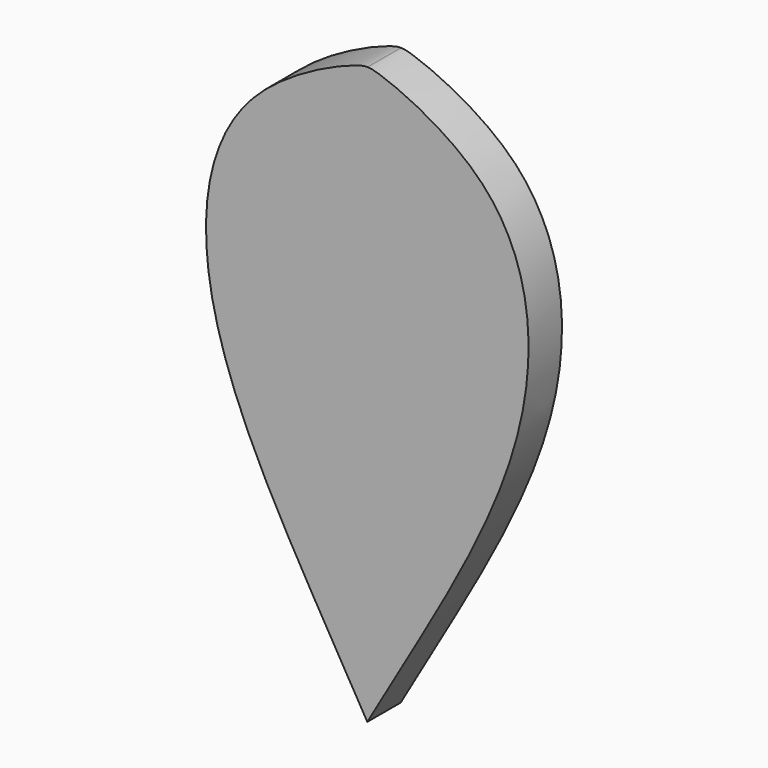
from build123d import *

# Parameters (mm, degrees)
F1_DEPTH = 5


with BuildPart() as f1:
    # F0 (on Front) → F1 (new body)
    with BuildSketch(Plane.XZ):
        with BuildLine():
            add(Edge.make_bspline(
                [(0, 0), (-7.8883632072, 13.8003130558), (-21.7462386942, 35.0909967896), (-18.519377881, 62.5951900227), (-0.8446341959, 69.1773688938), (-0.0343544445, 68.9731165883)],
                knots=[0, 0, 0, 0, 0.4098329947, 0.7231046582, 0.9651145636, 0.9651145636, 0.9651145636, 0.9651145636], degree=3))
            add(Edge.make_bspline(
                [(0, 0), (7.8883632072, 13.8003130558), (21.7462386942, 35.0909967896), (18.519377881, 62.5951900227), (0.8446341959, 69.1773688938), (0.0343544445, 68.9731165883)],
                knots=[0, 0, 0, 0, 0.4098329947, 0.7231046582, 0.9651145636, 0.9651145636, 0.9651145636, 0.9651145636], degree=3))
            add(Edge.make_bspline(
                [(0.0343544445, 68.9731165883), (0.0210221116, 68.9697558234), (0.0095559332, 68.9655630988), (0, 68.960532546)],
                knots=[0.9651145636, 0.9651145636, 0.9651145636, 0.9651145636, 0.9690965916, 0.9690965916, 0.9690965916, 0.9690965916], degree=3))
            add(Edge.make_bspline(
                [(-0.0343544445, 68.9731165883), (-0.0210221116, 68.9697558234), (-0.0095559332, 68.9655630988), (0, 68.960532546)],
                knots=[0.9651145636, 0.9651145636, 0.9651145636, 0.9651145636, 0.9690965916, 0.9690965916, 0.9690965916, 0.9690965916], degree=3))
        make_face()
        with BuildLine():
            add(Edge.make_bspline(
                [(0, 68.960532546), (-0.0741609324, 68.9214918294), (-0.033270113, 68.8319897358), (0, 68.7220096588)],
                knots=[0.9690965916, 0.9690965916, 0.9690965916, 0.9690965916, 1, 1, 1, 1], degree=3))
            add(Edge.make_bspline(
                [(0, 68.960532546), (0.0741609324, 68.9214918294), (0.033270113, 68.8319897358), (0, 68.7220096588)],
                knots=[0.9690965916, 0.9690965916, 0.9690965916, 0.9690965916, 1, 1, 1, 1], degree=3))
        make_face(mode=Mode.SUBTRACT)
        with BuildLine():
            add(Edge.make_bspline(
                [(0, 68.960532546), (0.0741609324, 68.9214918294), (0.033270113, 68.8319897358), (0, 68.7220096588)],
                knots=[0.9690965916, 0.9690965916, 0.9690965916, 0.9690965916, 1, 1, 1, 1], degree=3))
            add(Edge.make_bspline(
                [(0, 68.960532546), (-0.0741609324, 68.9214918294), (-0.033270113, 68.8319897358), (0, 68.7220096588)],
                knots=[0.9690965916, 0.9690965916, 0.9690965916, 0.9690965916, 1, 1, 1, 1], degree=3))
        make_face()
        with BuildLine():
            Line((0.0343544445, 68.9731165883), (-0.0343544445, 68.9731165883))
            add(Edge.make_bspline(
                [(-0.0343544445, 68.9731165883), (-0.0210221116, 68.9697558234), (-0.0095559332, 68.9655630988), (0, 68.960532546)],
                knots=[0.9651145636, 0.9651145636, 0.9651145636, 0.9651145636, 0.9690965916, 0.9690965916, 0.9690965916, 0.9690965916], degree=3))
            add(Edge.make_bspline(
                [(0.0343544445, 68.9731165883), (0.0210221116, 68.9697558234), (0.0095559332, 68.9655630988), (0, 68.960532546)],
                knots=[0.9651145636, 0.9651145636, 0.9651145636, 0.9651145636, 0.9690965916, 0.9690965916, 0.9690965916, 0.9690965916], degree=3))
        make_face()
    extrude(amount=F1_DEPTH)


solid = f1.part
